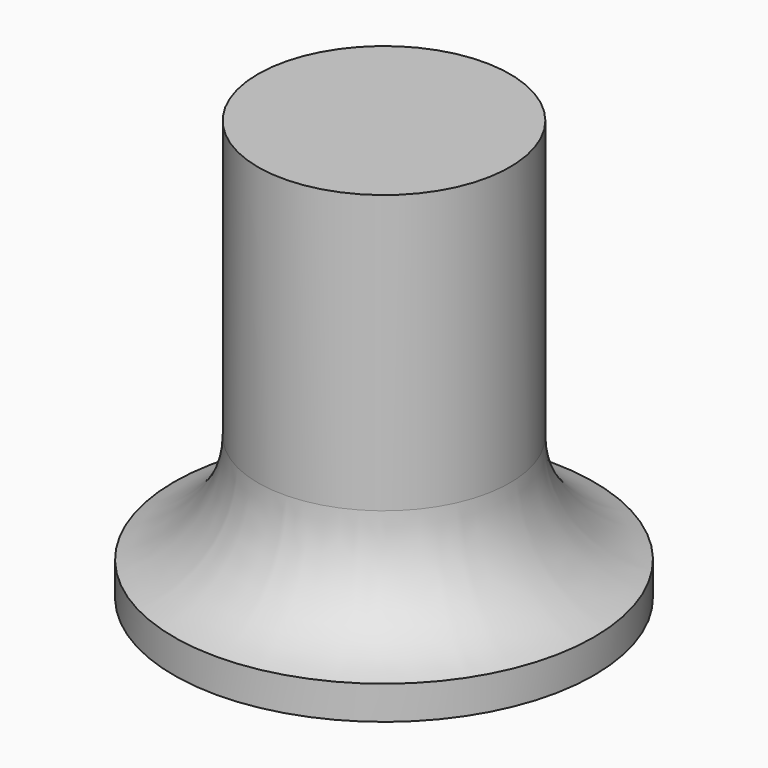
from build123d import *

# Parameters (mm, degrees)
F0_W = 9.525
F0_H = 1.524
F2_W = 5.715
F2_H = 19.05


# Not quite as in the source:
# - a fillet or chamfer that OpenCascade refuses, or shapes differently, is made with other operations: its cross-section is extruded or revolved along the edge and cut away or added


with BuildPart() as f1:
    # F0 (on Front) → F1 (revolve)
    with BuildSketch(Plane.XZ):
        with Locations((-4.7625, 0.762)):
            Rectangle(F0_W, F0_H)
    revolve(axis=Axis((0, 0, 0.762), (0, 0, 1)))

    # F2 (on Front) → F3 (revolve)
    with BuildSketch(Plane.XZ):
        with Locations((-2.8575, 9.525)):
            Rectangle(F2_W, F2_H)
    revolve(axis=Axis((0, 0, 9.525), (0, 0, 1)))

    # F4: fillet of radius 5.08 on 1 edges, made by hand

    # F4_s1 → F4_t2 (revolve)
    with BuildSketch(Plane.XZ):
        with BuildLine():
            ThreePointArc((-9.525, 1.524), (-6.7789073716, 3.3318368763), (-5.715, 6.4426888497))
            Line((-5.715, 6.4426888497), (-5.6134, 6.4426888497))
            Line((-5.6134, 6.4426888497), (-5.6134, 1.524))
            Line((-5.6134, 1.524), (-5.715, 1.4224))
            ThreePointArc((-5.715, 1.4224), (-7.62, 1.4224), (-9.4996, 1.425626223))
            Line((-9.4996, 1.425626223), (-9.525, 1.524))
        make_face()
    revolve(axis=Axis((0, 0, 1.524), (0, 0, -1)))


solid = f1.part
